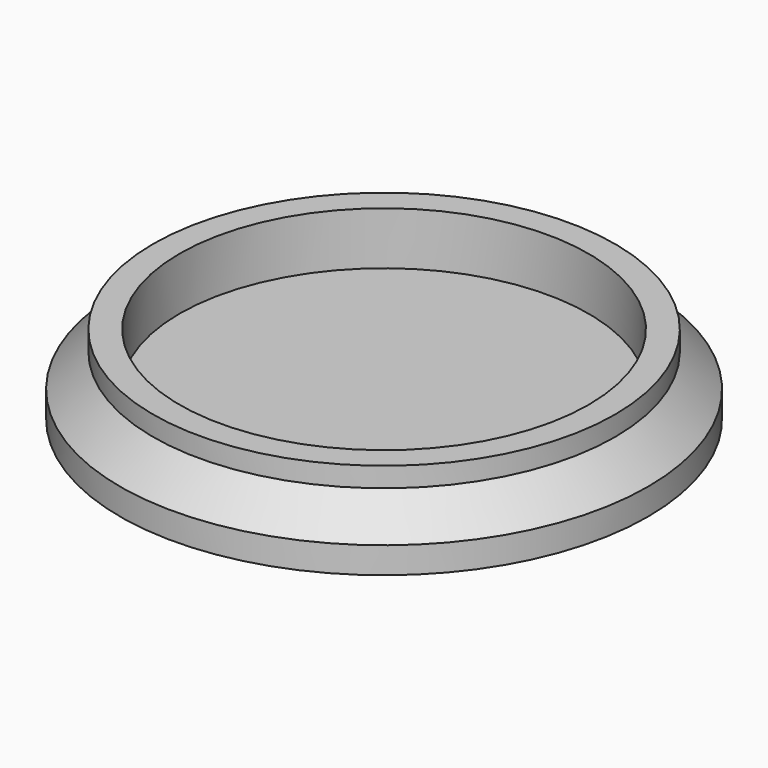
from build123d import *

# Parameters (mm, degrees)
F0_R     = 17.5
F0_R_2   = 15.5
F1_DEPTH = 6
F2_R     = 20
F3_DEPTH = 2
F4_SIZE  = 2.49999


# Not quite as in the source:
# - a fillet or chamfer is up to 0.001 mm smaller than in the source, because OpenCascade refuses the exact size


with BuildPart() as f1:
    # F0 (on Top) → F1 (new body)
    with BuildSketch(Plane.XY):
        Circle(F0_R)
        Circle(F0_R_2, mode=Mode.SUBTRACT)
    extrude(amount=F1_DEPTH)

    # F2 (on Top) → F3 (join)
    with BuildSketch(Plane.XY):
        Circle(F2_R)
    extrude(amount=F3_DEPTH)

    # F4 (size 2.5 in the source; OpenCascade refuses exactly that, so slightly less here)
    f4_edges = [f1.edges().sort_by_distance(p)[0] for p in [
        (-17.5, 0, 2),
    ]]
    chamfer(f4_edges, length=F4_SIZE)


solid = f1.part
